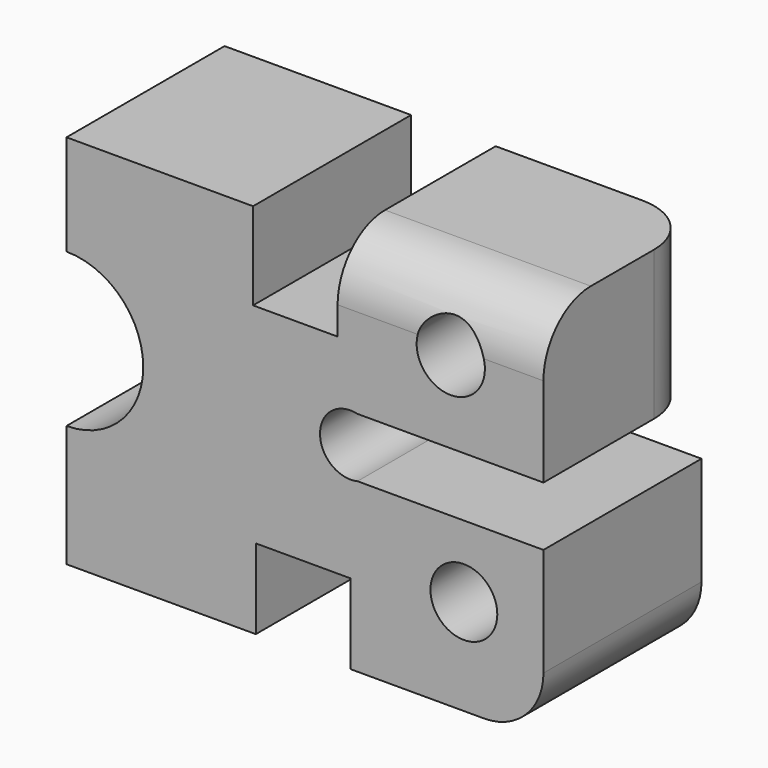
from build123d import *

# Parameters (mm, degrees)
F0_R        = 8.4621636151
F0_R_2      = 8.6410874337
F1_DEPTH    = 50
F4_T1_DEPTH = 125
F4_T3_DEPTH = 75.1791274175
F4_T8_DEPTH = 127.0995380357


# Not quite as in the source:
# - a fillet or chamfer that OpenCascade refuses, or shapes differently, is made with other operations: its cross-section is extruded or revolved along the edge and cut away or added
# - a feature of the source that left no trace in its solid (it failed there, or was rolled back) is left out


with BuildPart() as f1:
    # F0 (on Front) → F1 (new body)
    with BuildSketch(Plane.XZ):
        with BuildLine():
            Line((-12.9085844383, 52.6810027659), (-60.1237900555, 52.6810027659))
            Line((-60.1237900555, 52.6810027659), (-60.1237900555, 27.209569862))
            ThreePointArc((-60.1237900555, 27.209569862), (-40.7058920955, 7.7916719019), (-60.1237900555, -11.6262260581))
            Line((-60.1237900555, -11.6262260581), (-60.1237900555, -42.4471646547))
            Line((-60.1237900555, -42.4471646547), (-12.2108235955, -42.4471646547))
            Line((-12.2108235955, -42.4471646547), (-12.2108235955, -22.2120806575))
            Line((-12.2108235955, -22.2120806575), (11.7456596345, -22.2120806575))
            Line((11.7456596345, -22.2120806575), (11.7456596345, -42.4471646547))
            Line((11.7456596345, -42.4471646547), (60.588978231, -42.4471646547))
            Line((60.588978231, -42.4471646547), (60.588978231, 0))
            Line((60.588978231, 0), (13.5322010265, 0))
            ThreePointArc((13.5322010265, 0), (4.0349011674, 7.5009376742), (13.5322010265, 15.0018753484))
            Line((13.5322010265, 15.0018753484), (60.588978231, 15.0018753484))
            Line((60.588978231, 15.0018753484), (60.588978231, 52.6810027659))
            Line((60.588978231, 52.6810027659), (8.4894401953, 52.6810027659))
            Line((8.4894401953, 52.6810027659), (8.4894401953, 30.5852182209))
            Line((8.4894401953, 30.5852182209), (-12.9085844383, 30.5852182209))
            Line((-12.9085844383, 30.5852182209), (-12.9085844383, 52.6810027659))
        make_face()
        with Locations((40.4487065971, -18.1611850858)):
            Circle(F0_R, mode=Mode.SUBTRACT)
        with Locations((37.1295772493, 35.4981198907)):
            Circle(F0_R_2, mode=Mode.SUBTRACT)
    extrude(amount=F1_DEPTH)

    # F4: fillet of radius 15 on 3 edges, made by hand

    # F4_s2 → F4_t1 (cut)
    with BuildSketch(Plane.XZ.offset(-37.5)):
        with BuildLine():
            ThreePointArc((45.588978231, -42.4471646547), (56.1955799488, -38.0537663725), (60.588978231, -27.4471646547))
            Line((60.588978231, -27.4471646547), (60.588978231, -42.4471646547))
            Line((60.588978231, -42.4471646547), (45.588978231, -42.4471646547))
        make_face()
    extrude(amount=F4_T1_DEPTH, mode=Mode.SUBTRACT)

    # F4_s4 → F4_t3 (cut)
    with BuildSketch(Plane.XY.offset(15.0018753484)):
        with BuildLine():
            ThreePointArc((60.588978231, -15), (56.1955799488, -4.3933982822), (45.588978231, 0))
            Line((45.588978231, 0), (60.588978231, 0))
            Line((60.588978231, 0), (60.588978231, -15))
        make_face()
    extrude(amount=F4_T3_DEPTH, mode=Mode.SUBTRACT)


with BuildPart() as f4_tool6:
    # F4_s7 → F4_t8 (new body)
    with BuildSketch(Plane.YZ.offset(98.088978231)):
        with BuildLine():
            ThreePointArc((-35, 52.6810027659), (-45.6066017178, 48.2876044837), (-50, 37.6810027659))
            Line((-50, 37.6810027659), (-50, 52.6810027659))
            Line((-50, 52.6810027659), (-35, 52.6810027659))
        make_face()
    extrude(amount=-F4_T8_DEPTH)

    split(bisect_by=Plane.YZ.offset(-12.9085844383), keep=Keep.TOP)


with BuildPart() as f1_1:
    add(f1.part)

    # F4_t5: cut F4_tool6
    add(f4_tool6.part, mode=Mode.SUBTRACT)


solid = f1_1.part
